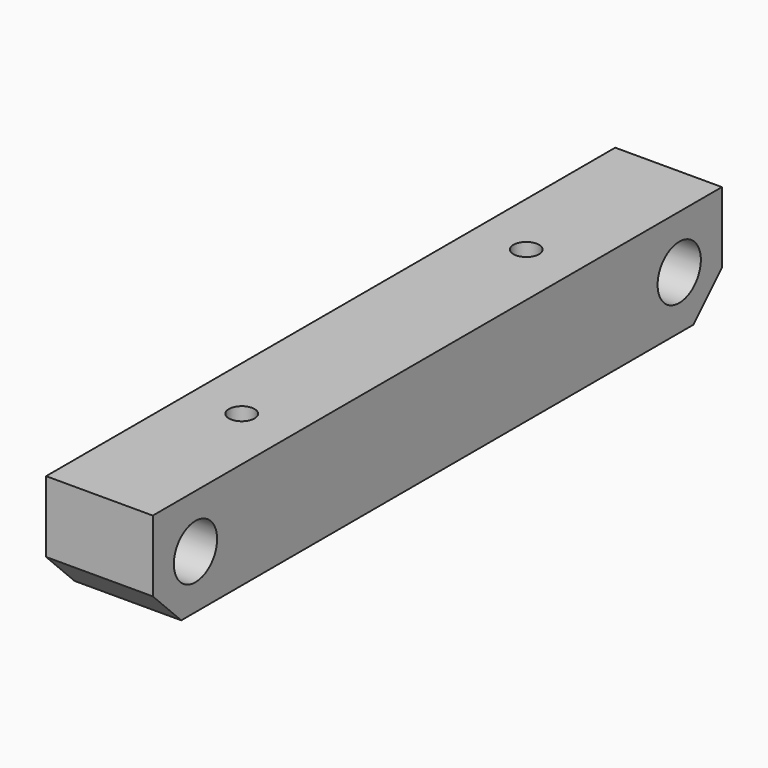
from build123d import *

# Parameters (mm, degrees)
F0_W     = 9.525
F0_H     = 63.5
F1_DEPTH = 9.525
F2_R     = 2.413
F3_DEPTH = 9.526
F4_R     = 1.143
F5_DEPTH = 6.35
F6_SIZE  = 3.175


# Not quite as in the source:
# - a pattern or mirror of a feature is missing from the dataset's text; its kind, count and spacing are read off the source's solid


with BuildPart() as f1:
    # F0 (on Top) → F1 (new body)
    with BuildSketch(Plane.XY):
        Rectangle(F0_W, F0_H)
    extrude(amount=F1_DEPTH)

    # F2 (on face) → F3 (cut, through all)
    with BuildSketch(Plane.YZ.offset(4.7625)):
        with Locations((-26.9875, 4.7625)):
            Circle(F2_R)
    f3 = extrude(amount=-F3_DEPTH, mode=Mode.SUBTRACT)

    # F3_copies: F3 across plane
    add(f3.mirror(Plane.ZX), mode=Mode.SUBTRACT)

    # F4 (on face) → F5 (cut)
    with BuildSketch(Plane.XY.offset(9.525)):
        with Locations((0, 15.875)):
            Circle(F4_R)
    f5 = extrude(amount=-F5_DEPTH, mode=Mode.SUBTRACT)

    # F5_copies: F5 across plane
    add(f5.mirror(Plane(origin=(0, 0, 0), x_dir=(0, 0, -1), z_dir=(0, -1, 0))), mode=Mode.SUBTRACT)

    # F6
    f6_edges = [f1.edges().sort_by_distance(p)[0] for p in [
        (0, -31.75, 0),
        (0, 31.75, 0),
    ]]
    chamfer(f6_edges, length=F6_SIZE)


solid = f1.part
